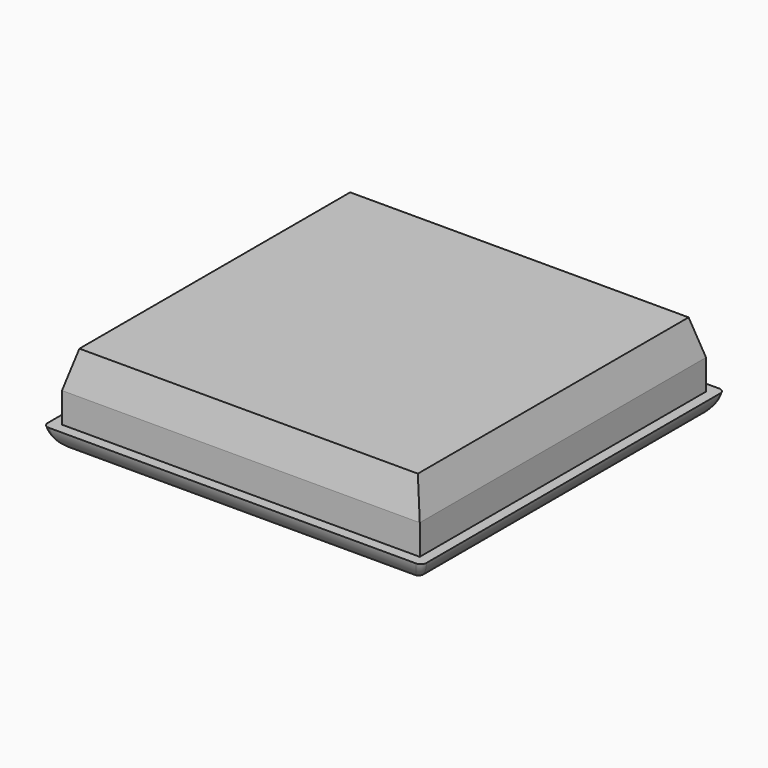
from build123d import *

# Parameters (mm, degrees)
F0_W        = 59.5
F0_H        = 59.5
F1_DEPTH    = 15
F0_W_2      = 63
F0_H_2      = 63
F2_DEPTH    = 4
F3_T1_DEPTH = 87.4948974279
F3_T3_DEPTH = 87.4948974279
F4_C1_SIZE2 = 1.6076951546
F4_C1_SIZE  = 6
F4_C2_SIZE2 = 1.6076951546
F4_C2_SIZE  = 6
F4_C3_SIZE2 = 1.6076951546
F4_C3_SIZE  = 6
F4_C4_SIZE2 = 1.6076951546
F4_C4_SIZE  = 6
F5_R        = 1


# Not quite as in the source:
# - a fillet or chamfer that OpenCascade refuses, or shapes differently, is made with other operations: its cross-section is extruded or revolved along the edge and cut away or added


with BuildPart() as f1:
    # F0 (on Top) → F1 (new body)
    with BuildSketch(Plane.XY):
        Rectangle(F0_W, F0_H)
    extrude(amount=F1_DEPTH)

    # F0 (on Top) → F2 (join)
    with BuildSketch(Plane.XY):
        Rectangle(F0_W_2, F0_H_2)
        Rectangle(F0_W, F0_H, mode=Mode.SUBTRACT)
    extrude(amount=F2_DEPTH)

    # F3: fillet of radius 5 on 4 edges, made by hand

    # F3_s2 → F3_t1 (cut)
    with BuildSketch(Plane.YZ.offset(-43.7474487139)):
        with BuildLine():
            ThreePointArc((-31.5, 4), (-29.7632981746, 1.1270166538), (-26.6010205144, 0))
            Line((-26.6010205144, 0), (-31.5, 0))
            Line((-31.5, 0), (-31.5, 4))
        make_face()
        with BuildLine():
            ThreePointArc((31.5, 4), (29.7632981746, 1.1270166538), (26.6010205144, 0))
            Line((26.6010205144, 0), (31.5, 0))
            Line((31.5, 0), (31.5, 4))
        make_face()
    extrude(amount=F3_T1_DEPTH, mode=Mode.SUBTRACT)

    # F3_s4 → F3_t3 (cut)
    with BuildSketch(Plane.XZ.offset(-43.7474487139)):
        with BuildLine():
            ThreePointArc((31.5, 4), (29.7632981746, 1.1270166538), (26.6010205144, 0))
            Line((26.6010205144, 0), (31.5, 0))
            Line((31.5, 0), (31.5, 4))
        make_face()
        with BuildLine():
            ThreePointArc((-31.5, 4), (-29.7632981746, 1.1270166538), (-26.6010205144, 0))
            Line((-26.6010205144, 0), (-31.5, 0))
            Line((-31.5, 0), (-31.5, 4))
        make_face()
    extrude(amount=F3_T3_DEPTH, mode=Mode.SUBTRACT)

    # F4: chamfer of 6 x 1.6076951546 on 4 edges, made by hand

    # F4_c1
    f4_c1_edges = [f1.edges().sort_by_distance(p)[0] for p in [
        (0, -29.75, 15),
    ]]
    f4_c1_side = f1.faces().sort_by_distance((0, -29.75, 14.9678460969))[0]
    chamfer(f4_c1_edges, length=F4_C1_SIZE, length2=F4_C1_SIZE2, reference=f4_c1_side)

    # F4_c2
    f4_c2_edges = [f1.edges().sort_by_distance(p)[0] for p in [
        (29.75, 0.8038475773, 15),
    ]]
    f4_c2_side = f1.faces().sort_by_distance((29.75, 0.8038475773, 14.9678460969))[0]
    chamfer(f4_c2_edges, length=F4_C2_SIZE, length2=F4_C2_SIZE2, reference=f4_c2_side)

    # F4_c3
    f4_c3_edges = [f1.edges().sort_by_distance(p)[0] for p in [
        (-0.8038475773, 29.75, 15),
    ]]
    f4_c3_side = f1.faces().sort_by_distance((-0.8038475773, 29.75, 14.9678460969))[0]
    chamfer(f4_c3_edges, length=F4_C3_SIZE, length2=F4_C3_SIZE2, reference=f4_c3_side)

    # F4_c4
    f4_c4_edges = [f1.edges().sort_by_distance(p)[0] for p in [
        (-29.75, 0, 15),
    ]]
    f4_c4_side = f1.faces().sort_by_distance((-29.75, 0, 14.9678460969))[0]
    chamfer(f4_c4_edges, length=F4_C4_SIZE, length2=F4_C4_SIZE2, reference=f4_c4_side)

    # F5
    f5_edges = [f1.edges().sort_by_distance(p)[0] for p in [
        (-29.517588, -29.517588, 0.938765),
        (-29.517588, 29.517588, 0.938765),
        (29.517588, 29.517588, 0.938765),
        (29.517588, -29.517588, 0.938765),
    ]]
    fillet(f5_edges, radius=F5_R)


solid = f1.part
